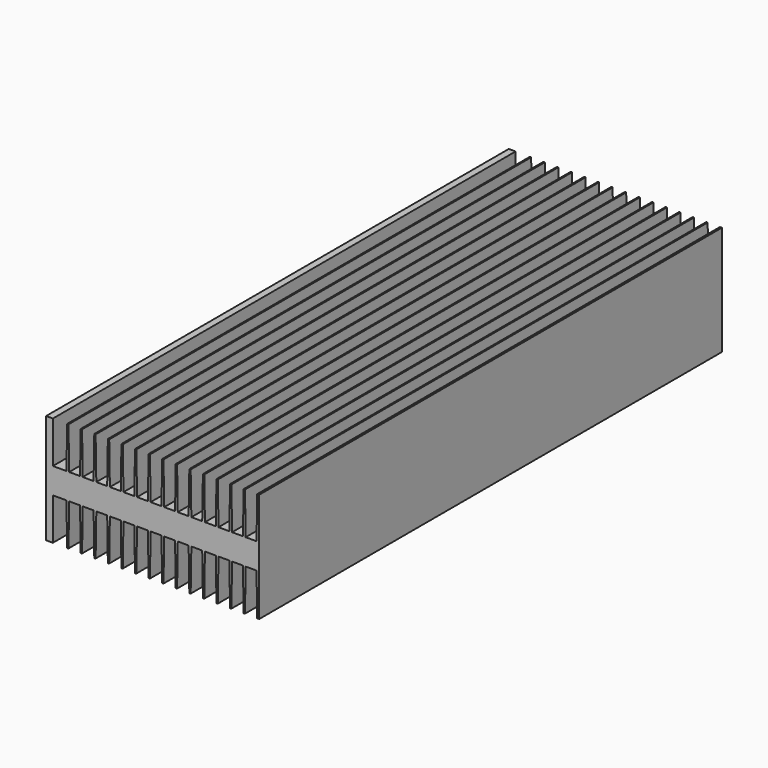
from build123d import *

# Parameters (mm, degrees)
F1_DEPTH = 426
F2_ANGLE = 180


with BuildPart() as f1:
    # F0 (on Front) → F1 (new body)
    with BuildSketch(Plane.XZ):
        with BuildLine():
            Line((8, 0), (0, 0))
            Line((0, 0), (-0.4980315916, 30.6787460424))
            ThreePointArc((-0.4980315916, 30.6787460424), (-0.5348260052, 30.764604049), (-0.6212699339, 30.8))
            Line((-0.6212699339, 30.8), (-1.5, 30.8))
            Line((-1.5, 30.8), (-2, 30.8))
            Line((-2, 30.8), (-2, -9.5))
            Line((-2, -9.5), (155, -9.5))
            Line((155, -9.5), (155, 30.8))
            Line((155, 30.8), (150, 30.8))
            Line((150, 30.8), (150, 0))
            Line((150, 0), (140, 0))
            Line((140, 0), (139.5019684084, 30.6787460424))
            ThreePointArc((139.5019684084, 30.6787460424), (139.4651739948, 30.764604049), (139.3787300661, 30.8))
            Line((139.3787300661, 30.8), (138.6212699339, 30.8))
            ThreePointArc((138.6212699339, 30.8), (138.5348260052, 30.764604049), (138.4980315916, 30.6787460424))
            Line((138.4980315916, 30.6787460424), (138, 0))
            Line((138, 0), (130, 0))
            Line((130, 0), (129.5019684084, 30.6787460424))
            ThreePointArc((129.5019684084, 30.6787460424), (129.4651739948, 30.764604049), (129.3787300661, 30.8))
            Line((129.3787300661, 30.8), (128.6212699339, 30.8))
            ThreePointArc((128.6212699339, 30.8), (128.5348260052, 30.764604049), (128.4980315916, 30.6787460424))
            Line((128.4980315916, 30.6787460424), (128, 0))
            Line((128, 0), (120, 0))
            Line((120, 0), (119.5019684084, 30.6787460424))
            ThreePointArc((119.5019684084, 30.6787460424), (119.4651739948, 30.764604049), (119.3787300661, 30.8))
            Line((119.3787300661, 30.8), (118.6212699339, 30.8))
            ThreePointArc((118.6212699339, 30.8), (118.5348260052, 30.764604049), (118.4980315916, 30.6787460424))
            Line((118.4980315916, 30.6787460424), (118, 0))
            Line((118, 0), (110, 0))
            Line((110, 0), (109.5019684084, 30.6787460424))
            ThreePointArc((109.5019684084, 30.6787460424), (109.4651739948, 30.764604049), (109.3787300661, 30.8))
            Line((109.3787300661, 30.8), (108.6212699339, 30.8))
            ThreePointArc((108.6212699339, 30.8), (108.5348260052, 30.764604049), (108.4980315916, 30.6787460424))
            Line((108.4980315916, 30.6787460424), (108, 0))
            Line((108, 0), (100, 0))
            Line((100, 0), (99.5019684084, 30.6787460424))
            ThreePointArc((99.5019684084, 30.6787460424), (99.4651739948, 30.764604049), (99.3787300661, 30.8))
            Line((99.3787300661, 30.8), (98.6212699339, 30.8))
            ThreePointArc((98.6212699339, 30.8), (98.5348260052, 30.764604049), (98.4980315916, 30.6787460424))
            Line((98.4980315916, 30.6787460424), (98, 0))
            Line((98, 0), (90, 0))
            Line((90, 0), (89.5019684084, 30.6787460424))
            ThreePointArc((89.5019684084, 30.6787460424), (89.4651739948, 30.764604049), (89.3787300661, 30.8))
            Line((89.3787300661, 30.8), (88.6212699339, 30.8))
            ThreePointArc((88.6212699339, 30.8), (88.5348260052, 30.764604049), (88.4980315916, 30.6787460424))
            Line((88.4980315916, 30.6787460424), (88, 0))
            Line((88, 0), (80, 0))
            Line((80, 0), (79.5019684084, 30.6787460424))
            ThreePointArc((79.5019684084, 30.6787460424), (79.4651739948, 30.764604049), (79.3787300661, 30.8))
            Line((79.3787300661, 30.8), (78.6212699339, 30.8))
            ThreePointArc((78.6212699339, 30.8), (78.5348260052, 30.764604049), (78.4980315916, 30.6787460424))
            Line((78.4980315916, 30.6787460424), (78, 0))
            Line((78, 0), (70, 0))
            Line((70, 0), (69.5019684084, 30.6787460424))
            ThreePointArc((69.5019684084, 30.6787460424), (69.4651739948, 30.764604049), (69.3787300661, 30.8))
            Line((69.3787300661, 30.8), (68.6212699339, 30.8))
            ThreePointArc((68.6212699339, 30.8), (68.5348260052, 30.764604049), (68.4980315916, 30.6787460424))
            Line((68.4980315916, 30.6787460424), (68, 0))
            Line((68, 0), (60, 0))
            Line((60, 0), (59.5019684084, 30.6787460424))
            ThreePointArc((59.5019684084, 30.6787460424), (59.4651739948, 30.764604049), (59.3787300661, 30.8))
            Line((59.3787300661, 30.8), (58.6212699339, 30.8))
            ThreePointArc((58.6212699339, 30.8), (58.5348260052, 30.764604049), (58.4980315916, 30.6787460424))
            Line((58.4980315916, 30.6787460424), (58, 0))
            Line((58, 0), (50, 0))
            Line((50, 0), (49.5019684084, 30.6787460424))
            ThreePointArc((49.5019684084, 30.6787460424), (49.4651739948, 30.764604049), (49.3787300661, 30.8))
            Line((49.3787300661, 30.8), (48.6212699339, 30.8))
            ThreePointArc((48.6212699339, 30.8), (48.5348260052, 30.764604049), (48.4980315916, 30.6787460424))
            Line((48.4980315916, 30.6787460424), (48, 0))
            Line((48, 0), (40, 0))
            Line((40, 0), (39.5019684084, 30.6787460424))
            ThreePointArc((39.5019684084, 30.6787460424), (39.4651739948, 30.764604049), (39.3787300661, 30.8))
            Line((39.3787300661, 30.8), (38.6212699339, 30.8))
            ThreePointArc((38.6212699339, 30.8), (38.5348260052, 30.764604049), (38.4980315916, 30.6787460424))
            Line((38.4980315916, 30.6787460424), (38, 0))
            Line((38, 0), (30, 0))
            Line((30, 0), (29.5019684084, 30.6787460424))
            ThreePointArc((29.5019684084, 30.6787460424), (29.4651739948, 30.764604049), (29.3787300661, 30.8))
            Line((29.3787300661, 30.8), (28.6212699339, 30.8))
            ThreePointArc((28.6212699339, 30.8), (28.5348260052, 30.764604049), (28.4980315916, 30.6787460424))
            Line((28.4980315916, 30.6787460424), (28, 0))
            Line((28, 0), (20, 0))
            Line((20, 0), (19.5019684084, 30.6787460424))
            ThreePointArc((19.5019684084, 30.6787460424), (19.4651739948, 30.764604049), (19.3787300661, 30.8))
            Line((19.3787300661, 30.8), (18.6212699339, 30.8))
            ThreePointArc((18.6212699339, 30.8), (18.5348260052, 30.764604049), (18.4980315916, 30.6787460424))
            Line((18.4980315916, 30.6787460424), (18, 0))
            Line((18, 0), (10, 0))
            Line((10, 0), (9.5019684084, 30.6787460424))
            ThreePointArc((9.5019684084, 30.6787460424), (9.4651739948, 30.764604049), (9.3787300661, 30.8))
            Line((9.3787300661, 30.8), (9, 30.8))
            Line((9, 30.8), (8.6212699339, 30.8))
            ThreePointArc((8.6212699339, 30.8), (8.5348260052, 30.764604049), (8.4980315916, 30.6787460424))
            Line((8.4980315916, 30.6787460424), (8, 0))
        make_face()
    extrude(amount=F1_DEPTH)


with BuildPart() as f1_1:
    # F2: moved
    add(f1.part.rotate(Axis((155, -213, -9.5), (0, 1, 0)), F2_ANGLE))


with BuildPart() as f1_2:
    # F3: moved
    add(f1_1.part.moved(Location((-179, -94, 509.5))))

    # F4: F1 across face


with BuildPart() as f1_3:
    add(f1_2.part)
    add(f1_2.part.mirror(Plane(origin=(54.5, -307, 500), x_dir=(1, 0, 0), z_dir=(0, 0, 1))))


solid = f1_3.part
